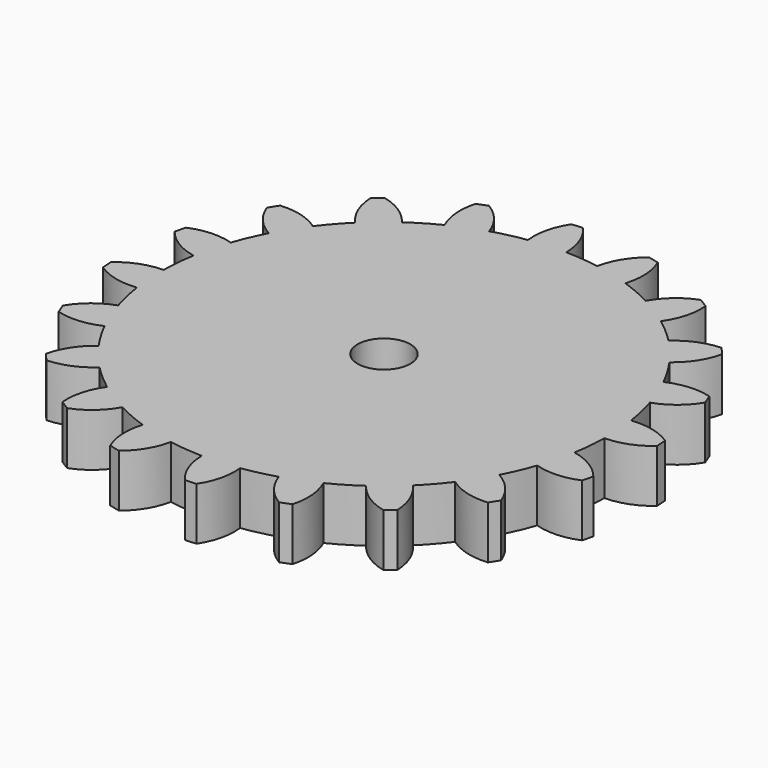
from build123d import *

# Parameters (mm, degrees)
F1_R     = 2.5
F2_DEPTH = 5


with BuildPart() as f2:
    # F1 (on Top) → F2 (new body)
    with BuildSketch(Plane.XY):
        with BuildLine():
            ThreePointArc((-3.1021413291, 20.9251505676), (-1.3835277337, 21.1085541454), (0.3443218548, 21.1510436991))
            ThreePointArc((0.3443218548, 21.1510436991), (-0.0428266044, 23.1934529579), (-1.1136971825, 24.9751812523))
            Line((-1.1136971825, 24.9751812523), (-2.1557459601, 24.906881767))
            ThreePointArc((-2.1557459601, 24.906881767), (-2.9848928822, 23.0006197463), (-3.1021413291, 20.9251505676))
        make_face()
        with BuildLine():
            ThreePointArc((21.1510436991, -0.3443218548), (21.1531455286, -0.1721666296), (21.1538461538, 0))
            ThreePointArc((21.1538461538, 0), (21.0965947839, 1.5552799183), (20.9251505676, 3.1021413291))
            ThreePointArc((20.9251505676, 3.1021413291), (20.6322413954, 4.668599587), (20.2222392411, 6.2085624081))
            ThreePointArc((20.2222392411, 6.2085624081), (19.6478943877, 7.8387150242), (18.9423864121, 9.4165388608))
            ThreePointArc((18.9423864121, 9.4165388608), (18.1797510125, 10.8158152824), (17.3139411096, 12.1537093248))
            ThreePointArc((17.3139411096, 12.1537093248), (16.2639618323, 13.5265942727), (15.1054094952, 14.8091799598))
            ThreePointArc((15.1054094952, 14.8091799598), (13.9476999348, 15.9043036197), (12.710833789, 16.909166493))
            ThreePointArc((12.710833789, 16.909166493), (11.2879993751, 17.8903962284), (9.7898098514, 18.7521953428))
            ThreePointArc((9.7898098514, 18.7521953428), (8.3503508081, 19.435967907), (6.8635014955, 20.0094366318))
            ThreePointArc((6.8635014955, 20.0094366318), (5.207088891, 20.5029615515), (3.5159154097, 20.8596151914))
            ThreePointArc((3.5159154097, 20.8596151914), (1.935611164, 21.0651042372), (0.3443218548, 21.1510436991))
            ThreePointArc((0.3443218548, 21.1510436991), (-1.3835277337, 21.1085541454), (-3.1021413291, 20.9251505676))
            ThreePointArc((-3.1021413291, 20.9251505676), (-4.668599587, 20.6322413954), (-6.2085624081, 20.2222392411))
            ThreePointArc((-6.2085624081, 20.2222392411), (-7.8387150242, 19.6478943877), (-9.4165388608, 18.9423864121))
            ThreePointArc((-9.4165388608, 18.9423864121), (-10.8158152824, 18.1797510125), (-12.1537093248, 17.3139411096))
            ThreePointArc((-12.1537093248, 17.3139411096), (-13.5265942727, 16.2639618323), (-14.8091799598, 15.1054094952))
            ThreePointArc((-14.8091799598, 15.1054094952), (-15.9043036197, 13.9476999348), (-16.909166493, 12.710833789))
            ThreePointArc((-16.909166493, 12.710833789), (-17.8903962284, 11.2879993751), (-18.7521953428, 9.7898098514))
            ThreePointArc((-18.7521953428, 9.7898098514), (-19.435967907, 8.3503508081), (-20.0094366318, 6.8635014955))
            ThreePointArc((-20.0094366318, 6.8635014955), (-20.5029615515, 5.207088891), (-20.8596151914, 3.5159154097))
            ThreePointArc((-20.8596151914, 3.5159154097), (-21.0651042372, 1.935611164), (-21.1510436991, 0.3443218548))
            ThreePointArc((-21.1510436991, 0.3443218548), (-21.1085541454, -1.3835277337), (-20.9251505676, -3.1021413291))
            ThreePointArc((-20.9251505676, -3.1021413291), (-20.6322413954, -4.668599587), (-20.2222392411, -6.2085624081))
            ThreePointArc((-20.2222392411, -6.2085624081), (-19.6478943877, -7.8387150242), (-18.9423864121, -9.4165388608))
            ThreePointArc((-18.9423864121, -9.4165388608), (-18.1797510125, -10.8158152824), (-17.3139411096, -12.1537093248))
            ThreePointArc((-17.3139411096, -12.1537093248), (-16.2639618323, -13.5265942727), (-15.1054094952, -14.8091799598))
            ThreePointArc((-15.1054094952, -14.8091799598), (-13.9476999348, -15.9043036197), (-12.710833789, -16.909166493))
            ThreePointArc((-12.710833789, -16.909166493), (-11.2879993751, -17.8903962284), (-9.7898098514, -18.7521953428))
            ThreePointArc((-9.7898098514, -18.7521953428), (-8.3503508081, -19.435967907), (-6.8635014955, -20.0094366318))
            ThreePointArc((-6.8635014955, -20.0094366318), (-5.207088891, -20.5029615515), (-3.5159154097, -20.8596151914))
            ThreePointArc((-3.5159154097, -20.8596151914), (-1.935611164, -21.0651042372), (-0.3443218548, -21.1510436991))
            ThreePointArc((-0.3443218548, -21.1510436991), (1.3835277337, -21.1085541454), (3.1021413291, -20.9251505676))
            ThreePointArc((3.1021413291, -20.9251505676), (4.668599587, -20.6322413954), (6.2085624081, -20.2222392411))
            ThreePointArc((6.2085624081, -20.2222392411), (7.8387150242, -19.6478943877), (9.4165388608, -18.9423864121))
            ThreePointArc((9.4165388608, -18.9423864121), (10.8158152824, -18.1797510125), (12.1537093248, -17.3139411096))
            ThreePointArc((12.1537093248, -17.3139411096), (13.5265942727, -16.2639618323), (14.8091799598, -15.1054094952))
            ThreePointArc((14.8091799598, -15.1054094952), (15.9043036197, -13.9476999348), (16.909166493, -12.710833789))
            ThreePointArc((16.909166493, -12.710833789), (17.8903962284, -11.2879993751), (18.7521953428, -9.7898098514))
            ThreePointArc((18.7521953428, -9.7898098514), (19.435967907, -8.3503508081), (20.0094366318, -6.8635014955))
            ThreePointArc((20.0094366318, -6.8635014955), (20.5029615515, -5.207088891), (20.8596151914, -3.5159154097))
            ThreePointArc((20.8596151914, -3.5159154097), (21.0651042372, -1.935611164), (21.1510436991, -0.3443218548))
        make_face()
        Circle(F1_R, mode=Mode.SUBTRACT)
        with BuildLine():
            ThreePointArc((-9.4165388608, 18.9423864121), (-7.8387150242, 19.6478943877), (-6.2085624081, 20.2222392411))
            ThreePointArc((-6.2085624081, 20.2222392411), (-7.2079016434, 22.0450504225), (-8.7769444072, 23.4086575197))
            Line((-8.7769444072, 23.4086575197), (-9.7468859857, 23.0216900679))
            ThreePointArc((-9.7468859857, 23.0216900679), (-9.9463842088, 20.9525066615), (-9.4165388608, 18.9423864121))
        make_face()
        with BuildLine():
            ThreePointArc((-14.8091799598, 15.1054094952), (-13.5265942727, 16.2639618323), (-12.1537093248, 17.3139411096))
            ThreePointArc((-12.1537093248, 17.3139411096), (-13.6674170492, 18.7387247548), (-15.5810431607, 19.5507312913))
            Line((-15.5810431607, 19.5507312913), (-16.3839329005, 18.8829749434))
            ThreePointArc((-16.3839329005, 18.8829749434), (-15.9342541485, 16.8534162401), (-14.8091799598, 15.1054094952))
        make_face()
        with BuildLine():
            ThreePointArc((-18.7521953428, 9.7898098514), (-17.8903962284, 11.2879993751), (-16.909166493, 12.710833789))
            ThreePointArc((-16.909166493, 12.710833789), (-18.7890704477, 13.5981221477), (-20.8599608501, 13.7790432662))
            Line((-20.8599608501, 13.7790432662), (-21.4172063094, 12.895862666))
            ThreePointArc((-21.4172063094, 12.895862666), (-20.3623682717, 11.1045960124), (-18.7521953428, 9.7898098514))
        make_face()
        with BuildLine():
            ThreePointArc((-20.8596151914, 3.5159154097), (-20.5029615515, 5.207088891), (-20.0094366318, 6.8635014955))
            ThreePointArc((-20.0094366318, 6.8635014955), (-22.0715187196, 7.1264406011), (-24.0969602317, 6.6585664819))
            Line((-24.0969602317, 6.6585664819), (-24.3540143423, 5.6464135001))
            ThreePointArc((-24.3540143423, 5.6464135001), (-22.7972719155, 4.2687805567), (-20.8596151914, 3.5159154097))
        make_face()
        with BuildLine():
            ThreePointArc((-20.9251505676, -3.1021413291), (-21.1085541454, -1.3835277337), (-21.1510436991, 0.3443218548))
            ThreePointArc((-21.1510436991, 0.3443218548), (-23.1934529579, -0.0428266044), (-24.9751812523, -1.1136971825))
            Line((-24.9751812523, -1.1136971825), (-24.906881767, -2.1557459601))
            ThreePointArc((-24.906881767, -2.1557459601), (-23.0006197463, -2.9848928822), (-20.9251505676, -3.1021413291))
        make_face()
        with BuildLine():
            ThreePointArc((-23.0216900679, -9.7468859857), (-20.9525066615, -9.9463842088), (-18.9423864121, -9.4165388608))
            ThreePointArc((-18.9423864121, -9.4165388608), (-19.6478943877, -7.8387150242), (-20.2222392411, -6.2085624081))
            ThreePointArc((-20.2222392411, -6.2085624081), (-22.0450504225, -7.2079016434), (-23.4086575197, -8.7769444072))
            Line((-23.4086575197, -8.7769444072), (-23.0216900679, -9.7468859857))
        make_face()
        with BuildLine():
            ThreePointArc((-18.8829749434, -16.3839329005), (-16.8534162401, -15.9342541485), (-15.1054094952, -14.8091799598))
            ThreePointArc((-15.1054094952, -14.8091799598), (-16.2639618323, -13.5265942727), (-17.3139411096, -12.1537093248))
            ThreePointArc((-17.3139411096, -12.1537093248), (-18.7387247548, -13.6674170492), (-19.5507312913, -15.5810431607))
            Line((-19.5507312913, -15.5810431607), (-18.8829749434, -16.3839329005))
        make_face()
        with BuildLine():
            ThreePointArc((-12.895862666, -21.4172063094), (-11.1045960124, -20.3623682717), (-9.7898098514, -18.7521953428))
            ThreePointArc((-9.7898098514, -18.7521953428), (-11.2879993751, -17.8903962284), (-12.710833789, -16.909166493))
            ThreePointArc((-12.710833789, -16.909166493), (-13.5981221477, -18.7890704477), (-13.7790432662, -20.8599608501))
            Line((-13.7790432662, -20.8599608501), (-12.895862666, -21.4172063094))
        make_face()
        with BuildLine():
            ThreePointArc((-5.6464135001, -24.3540143423), (-4.2687805567, -22.7972719155), (-3.5159154097, -20.8596151914))
            ThreePointArc((-3.5159154097, -20.8596151914), (-5.207088891, -20.5029615515), (-6.8635014955, -20.0094366318))
            ThreePointArc((-6.8635014955, -20.0094366318), (-7.1264406011, -22.0715187196), (-6.6585664819, -24.0969602317))
            Line((-6.6585664819, -24.0969602317), (-5.6464135001, -24.3540143423))
        make_face()
        with BuildLine():
            ThreePointArc((2.1557459601, -24.906881767), (2.9848928822, -23.0006197463), (3.1021413291, -20.9251505676))
            ThreePointArc((3.1021413291, -20.9251505676), (1.3835277337, -21.1085541454), (-0.3443218548, -21.1510436991))
            ThreePointArc((-0.3443218548, -21.1510436991), (0.0428266044, -23.1934529579), (1.1136971825, -24.9751812523))
            Line((1.1136971825, -24.9751812523), (2.1557459601, -24.906881767))
        make_face()
        with BuildLine():
            ThreePointArc((9.7468859857, -23.0216900679), (9.9463842088, -20.9525066615), (9.4165388608, -18.9423864121))
            ThreePointArc((9.4165388608, -18.9423864121), (7.8387150242, -19.6478943877), (6.2085624081, -20.2222392411))
            ThreePointArc((6.2085624081, -20.2222392411), (7.2079016434, -22.0450504225), (8.7769444072, -23.4086575197))
            Line((8.7769444072, -23.4086575197), (9.7468859857, -23.0216900679))
        make_face()
        with BuildLine():
            ThreePointArc((16.3839329005, -18.8829749434), (15.9342541485, -16.8534162401), (14.8091799598, -15.1054094952))
            ThreePointArc((14.8091799598, -15.1054094952), (13.5265942727, -16.2639618323), (12.1537093248, -17.3139411096))
            ThreePointArc((12.1537093248, -17.3139411096), (13.6674170492, -18.7387247548), (15.5810431607, -19.5507312913))
            Line((15.5810431607, -19.5507312913), (16.3839329005, -18.8829749434))
        make_face()
        with BuildLine():
            ThreePointArc((21.4172063094, -12.895862666), (20.3623682717, -11.1045960124), (18.7521953428, -9.7898098514))
            ThreePointArc((18.7521953428, -9.7898098514), (17.8903962284, -11.2879993751), (16.909166493, -12.710833789))
            ThreePointArc((16.909166493, -12.710833789), (18.7890704477, -13.5981221477), (20.8599608501, -13.7790432662))
            Line((20.8599608501, -13.7790432662), (21.4172063094, -12.895862666))
        make_face()
        with BuildLine():
            ThreePointArc((24.3540143423, -5.6464135001), (22.7972719155, -4.2687805567), (20.8596151914, -3.5159154097))
            ThreePointArc((20.8596151914, -3.5159154097), (20.5029615515, -5.207088891), (20.0094366318, -6.8635014955))
            ThreePointArc((20.0094366318, -6.8635014955), (22.0715187196, -7.1264406011), (24.0969602317, -6.6585664819))
            Line((24.0969602317, -6.6585664819), (24.3540143423, -5.6464135001))
        make_face()
        with BuildLine():
            ThreePointArc((20.9251505676, 3.1021413291), (21.0965947839, 1.5552799183), (21.1538461538, 0))
            ThreePointArc((21.1538461538, 0), (21.1531455286, -0.1721666296), (21.1510436991, -0.3443218548))
            ThreePointArc((21.1510436991, -0.3443218548), (23.1934529579, 0.0428266044), (24.9751812523, 1.1136971825))
            Line((24.9751812523, 1.1136971825), (24.906881767, 2.1557459601))
            ThreePointArc((24.906881767, 2.1557459601), (23.0006197463, 2.9848928822), (20.9251505676, 3.1021413291))
        make_face()
        with BuildLine():
            ThreePointArc((18.9423864121, 9.4165388608), (19.6478943877, 7.8387150242), (20.2222392411, 6.2085624081))
            ThreePointArc((20.2222392411, 6.2085624081), (22.0450504225, 7.2079016434), (23.4086575197, 8.7769444072))
            Line((23.4086575197, 8.7769444072), (23.0216900679, 9.7468859857))
            ThreePointArc((23.0216900679, 9.7468859857), (20.9525066615, 9.9463842088), (18.9423864121, 9.4165388608))
        make_face()
        with BuildLine():
            ThreePointArc((15.1054094952, 14.8091799598), (16.2639618323, 13.5265942727), (17.3139411096, 12.1537093248))
            ThreePointArc((17.3139411096, 12.1537093248), (18.7387247548, 13.6674170492), (19.5507312913, 15.5810431607))
            Line((19.5507312913, 15.5810431607), (18.8829749434, 16.3839329005))
            ThreePointArc((18.8829749434, 16.3839329005), (16.8534162401, 15.9342541485), (15.1054094952, 14.8091799598))
        make_face()
        with BuildLine():
            ThreePointArc((9.7898098514, 18.7521953428), (11.2879993751, 17.8903962284), (12.710833789, 16.909166493))
            ThreePointArc((12.710833789, 16.909166493), (13.5981221477, 18.7890704477), (13.7790432662, 20.8599608501))
            Line((13.7790432662, 20.8599608501), (12.895862666, 21.4172063094))
            ThreePointArc((12.895862666, 21.4172063094), (11.1045960124, 20.3623682717), (9.7898098514, 18.7521953428))
        make_face()
        with BuildLine():
            ThreePointArc((3.5159154097, 20.8596151914), (5.207088891, 20.5029615515), (6.8635014955, 20.0094366318))
            ThreePointArc((6.8635014955, 20.0094366318), (7.1264406011, 22.0715187196), (6.6585664819, 24.0969602317))
            Line((6.6585664819, 24.0969602317), (5.6464135001, 24.3540143423))
            ThreePointArc((5.6464135001, 24.3540143423), (4.2687805567, 22.7972719155), (3.5159154097, 20.8596151914))
        make_face()
    extrude(amount=F2_DEPTH)


solid = f2.part
